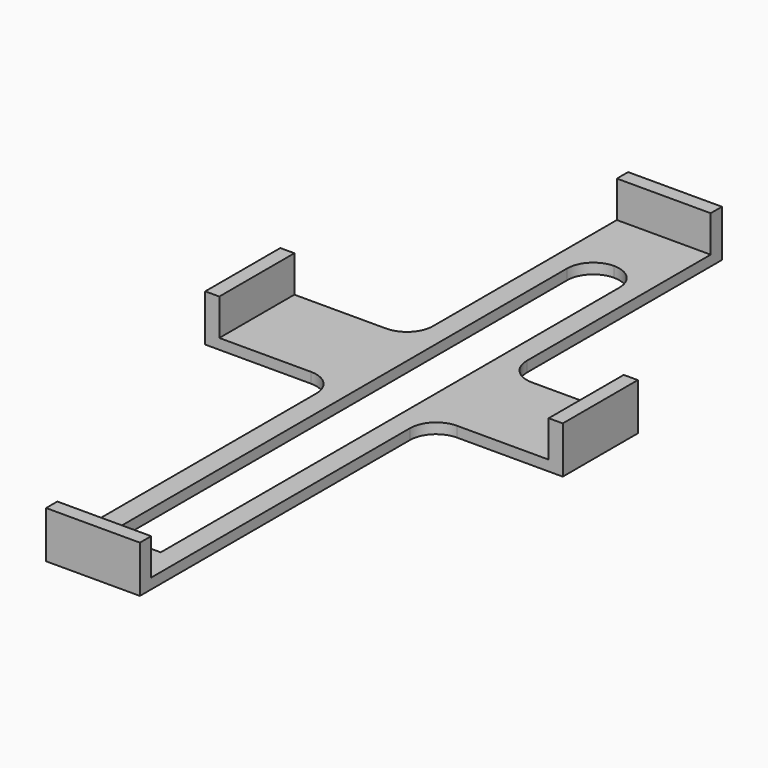
from build123d import *

# Parameters (mm, degrees)
F0_W     = 10
F0_H     = 115
F0_W_2   = 25.3
F0_H_2   = 18
F1_DEPTH = 2
F3_W     = 2.7
F3_H     = 18
F3_W_2   = 18
F3_H_2   = 2.7
F4_DEPTH = 7
F5_R     = 4.99999


# Not quite as in the source:
# - a fillet or chamfer is up to 0.001 mm smaller than in the source, because OpenCascade refuses the exact size


with BuildPart() as f1:
    # F0 (on Top) → F1 (new body)
    with BuildSketch(Plane.XY):
        Polygon((9, 135.3739356415), (-9, 135.3739356415), (-9, 83.5739356415), (-9, 65.5739356415), (-9, -4.2260643585), (9, -4.2260643585), (9, 65.5739356415), (9, 83.5739356415), align=None)
        with Locations((0, 63.2739356415)):
            Rectangle(F0_W, F0_H, mode=Mode.SUBTRACT)
        with Locations((-21.65, 74.5739356415)):
            Rectangle(F0_W_2, F0_H_2)
        with Locations((21.65, 74.5739356415)):
            Rectangle(F0_W_2, F0_H_2)
    extrude(amount=F1_DEPTH)

    # F3 (on face) → F4 (join)
    with BuildSketch(Plane.XY.offset(2)):
        with Locations((-32.95, 74.5739356415)):
            Rectangle(F3_W, F3_H)
        with Locations((32.95, 74.5739356415)):
            Rectangle(F3_W, F3_H)
        with Locations((0, 134.0239356415)):
            Rectangle(F3_W_2, F3_H_2)
        with Locations((0, -2.8760643585)):
            Rectangle(F3_W_2, F3_H_2)
    extrude(amount=F4_DEPTH)

    # F5 (radius 5 in the source; OpenCascade refuses exactly that, so slightly less here)
    f5_edges = [f1.edges().sort_by_distance(p)[0] for p in [
        (-9, 65.573936, 1),
        (9, 65.573936, 1),
        (9, 83.573936, 1),
        (-9, 83.573936, 1),
        (-5, 120.773936, 1),
        (5, 120.773936, 1),
    ]]
    fillet(f5_edges, radius=F5_R)


solid = f1.part
